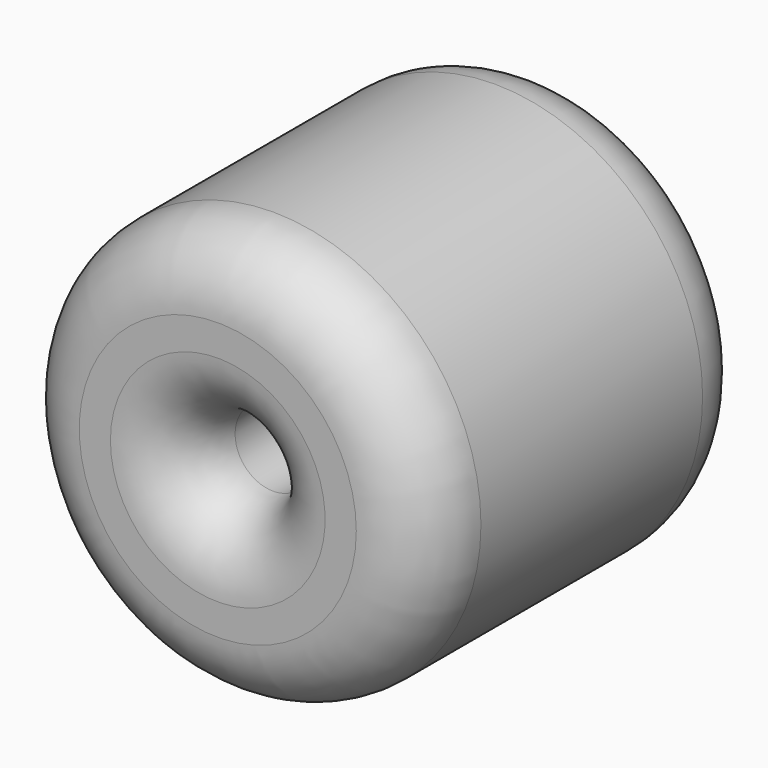
from build123d import *

# Parameters (mm, degrees)
F0_R     = 60
F1_DEPTH = 120
F3_D     = 22
F4_R     = 20


with BuildPart() as f1:
    # F0 (on Front) → F1 (new body)
    with BuildSketch(Plane.XZ):
        Circle(F0_R)
    extrude(amount=F1_DEPTH)

    # F3 (through all)
    with Locations(Plane.XZ.offset(120)):
        with Locations((0, 0)):
            Hole(F3_D / 2)

    # F4
    f4_edges = [f1.edges().sort_by_distance(p)[0] for p in [
        (60, -60, 0),
        (-60, 0, 0),
        (-60, -120, 0),
        (-11, 0, 0),
        (-11, -120, 0),
    ]]
    fillet(f4_edges, radius=F4_R)


solid = f1.part
